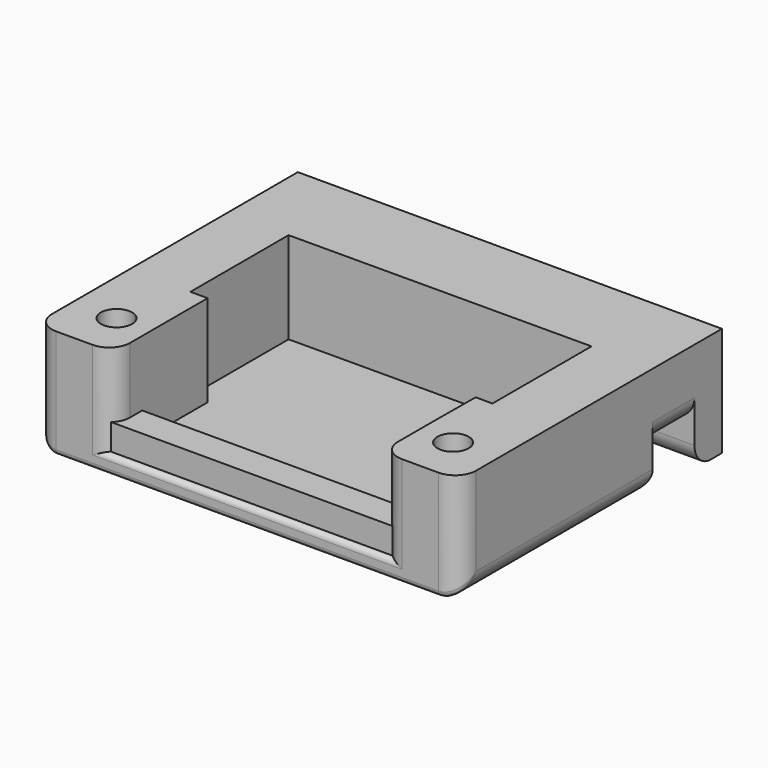
from build123d import *

# Parameters (mm, degrees)
F0_W           = 40.7
F0_H           = 23.2
F0_H_2         = 5
F0_H_3         = 1.8
F1_DEPTH       = 10.5
F2_D           = 3
F2_CBORE_D     = 6
F2_CBORE_DEPTH = 5
F3_D           = 3
F3_CBORE_D     = 6
F3_CBORE_DEPTH = 5
F4_DEPTH       = 4
F6_DEPTH       = 8.8
F7_T1_DEPTH    = 13.8
F7_T3_DEPTH    = 20.5
F7_T5_DEPTH    = 33.2
F7_T7_DEPTH    = 50.6498743711
F7_T9_DEPTH    = 50.7
F7_T11_DEPTH   = 5
F8_R           = 0.5
F10_DEPTH      = 2.5
F11_DEPTH      = 1.5


# Not quite as in the source:
# - a fillet or chamfer that OpenCascade refuses, or shapes differently, is made with other operations: its cross-section is extruded or revolved along the edge and cut away or added


with BuildPart() as f1:
    # F0 (on Top) → F1 (new body)
    with BuildSketch(Plane.XY):
        with Locations((0, -3.4)):
            Rectangle(F0_W, F0_H)
        with Locations((0, 10.7)):
            Rectangle(F0_W, F0_H_2)
        with Locations((0, 14.1)):
            Rectangle(F0_W, F0_H_3)
    extrude(amount=F1_DEPTH)

    # F2 (through all)
    with Locations(Plane(origin=(0, 0, 0), x_dir=(1, 0, 0), z_dir=(0, 0, -1))):
        with Locations((-16.15, 10.5)):
            CounterBoreHole(F2_D / 2, F2_CBORE_D / 2, F2_CBORE_DEPTH)

    # F3 (through all)
    with Locations(Plane(origin=(0, 0, 0), x_dir=(1, 0, 0), z_dir=(0, 0, -1))):
        with Locations((16.15, 10.5)):
            CounterBoreHole(F3_D / 2, F3_CBORE_D / 2, F3_CBORE_DEPTH)

    # F0 (on Top) → F4 (cut)
    with BuildSketch(Plane.XY):
        with Locations((0, 10.7)):
            Rectangle(F0_W, F0_H_2)
    extrude(amount=F4_DEPTH, mode=Mode.SUBTRACT)

    # F5 (on face) → F6 (cut)
    with BuildSketch(Plane.XY.offset(10.5)):
        Polygon((-12.85, -3.7), (-12.85, -8.6720474064), (-12.85, -15), (12.85, -15), (12.85, -8.5788490251), (12.886153895, -3.7037077804), (14.5, -3.7156760127), (14.5, 8.1671951339), (-14.5, 8.0755921081), (-14.5, -3.7), align=None)
    extrude(amount=-F6_DEPTH, mode=Mode.SUBTRACT)

    # F7: fillet of radius 2 on 10 edges, made by hand

    # F7_s2 → F7_t1 (cut)
    with BuildSketch(Plane.XY.offset(1.7)):
        with BuildLine():
            ThreePointArc((-14.85, -15), (-13.4357864376, -14.4142135624), (-12.85, -13))
            Line((-12.85, -13), (-12.85, -15))
            Line((-12.85, -15), (-14.85, -15))
        make_face()
        with BuildLine():
            ThreePointArc((14.85, -15), (13.4357864376, -14.4142135624), (12.85, -13))
            Line((12.85, -13), (12.85, -15))
            Line((12.85, -15), (14.85, -15))
        make_face()
    extrude(amount=F7_T1_DEPTH, mode=Mode.SUBTRACT)

    # F7_s4 → F7_t3 (cut)
    with BuildSketch(Plane.XY.offset(-5)):
        with BuildLine():
            ThreePointArc((-18.35, -15), (-19.7642135624, -14.4142135624), (-20.35, -13))
            Line((-20.35, -13), (-20.35, -15))
            Line((-20.35, -15), (-18.35, -15))
        make_face()
        with BuildLine():
            ThreePointArc((18.35, -15), (19.7642135624, -14.4142135624), (20.35, -13))
            Line((20.35, -13), (20.35, -15))
            Line((20.35, -15), (18.35, -15))
        make_face()
    extrude(amount=F7_T3_DEPTH, mode=Mode.SUBTRACT)

    # F7_s6 → F7_t5 (cut)
    with BuildSketch(Plane.XZ.offset(-13.2)):
        with BuildLine():
            ThreePointArc((-18.35, 0), (-19.7642135624, 0.5857864376), (-20.35, 2))
            Line((-20.35, 2), (-20.35, 0))
            Line((-20.35, 0), (-18.35, 0))
        make_face()
        with BuildLine():
            ThreePointArc((18.35, 0), (19.7642135624, 0.5857864376), (20.35, 2))
            Line((20.35, 2), (20.35, 0))
            Line((20.35, 0), (18.35, 0))
        make_face()
    extrude(amount=F7_T5_DEPTH, mode=Mode.SUBTRACT)

    # F7_s8 → F7_t7 (cut)
    with BuildSketch(Plane.YZ.offset(-25.3249371855)):
        with BuildLine():
            ThreePointArc((13.2, 1.9899748742), (13.7167603026, 0.6483340877), (15, 0))
            Line((15, 0), (13.2, 0))
            Line((13.2, 0), (13.2, 1.9899748742))
        make_face()
    extrude(amount=F7_T7_DEPTH, mode=Mode.SUBTRACT)

    # F7_s10 → F7_t9 (cut)
    with BuildSketch(Plane.YZ.offset(-25.35)):
        with BuildLine():
            ThreePointArc((6.2, 0), (7.6142135624, 0.5857864376), (8.2, 2))
            Line((8.2, 2), (8.2, 0))
            Line((8.2, 0), (6.2, 0))
        make_face()
    extrude(amount=F7_T9_DEPTH, mode=Mode.SUBTRACT)

    # F7_s12 → F7_t11 (cut)
    with BuildSketch(Plane.XZ.offset(-13.2)):
        with BuildLine():
            ThreePointArc((20.35, 6), (19.7642135624, 4.5857864376), (18.35, 4))
            Line((18.35, 4), (20.35, 4))
            Line((20.35, 4), (20.35, 6))
        make_face()
        with BuildLine():
            ThreePointArc((-20.35, 6), (-19.7642135624, 4.5857864376), (-18.35, 4))
            Line((-18.35, 4), (-20.35, 4))
            Line((-20.35, 4), (-20.35, 6))
        make_face()
    extrude(amount=F7_T11_DEPTH, mode=Mode.SUBTRACT)

    # F8
    f8_edges = [f1.edges().sort_by_distance(p)[0] for p in [
        (0, -15, 0),
        (0, -15, 1.7),
        (-19.764214, -14.414214, 0.585786),
        (19.764214, -14.414214, 0.585786),
    ]]
    fillet(f8_edges, radius=F8_R)

    # F9 (on face) → F10 (join)
    with BuildSketch(Plane.XY.offset(1.7)):
        with BuildLine():
            Line((12.85, -11.5439696237), (-12.85, -11.5439696237))
            Line((-12.85, -11.5439696237), (-12.85, -13))
            ThreePointArc((-12.85, -13), (-13.0181614416, -13.802725044), (-13.4943674962, -14.4704626873))
            Line((-13.4943674962, -14.4704626873), (13.4943674962, -14.4704626873))
            ThreePointArc((13.4943674962, -14.4704626873), (13.0181614416, -13.802725044), (12.85, -13))
            Line((12.85, -13), (12.85, -11.5439696237))
        make_face()
    extrude(amount=F10_DEPTH)

    # F11 (add): a face of the model
    f11_faces = [f1.faces().sort_by_distance(p)[0] for p in [
        (0, 15, 5.25),
    ]]
    extrude(f11_faces, amount=F11_DEPTH)


solid = f1.part
